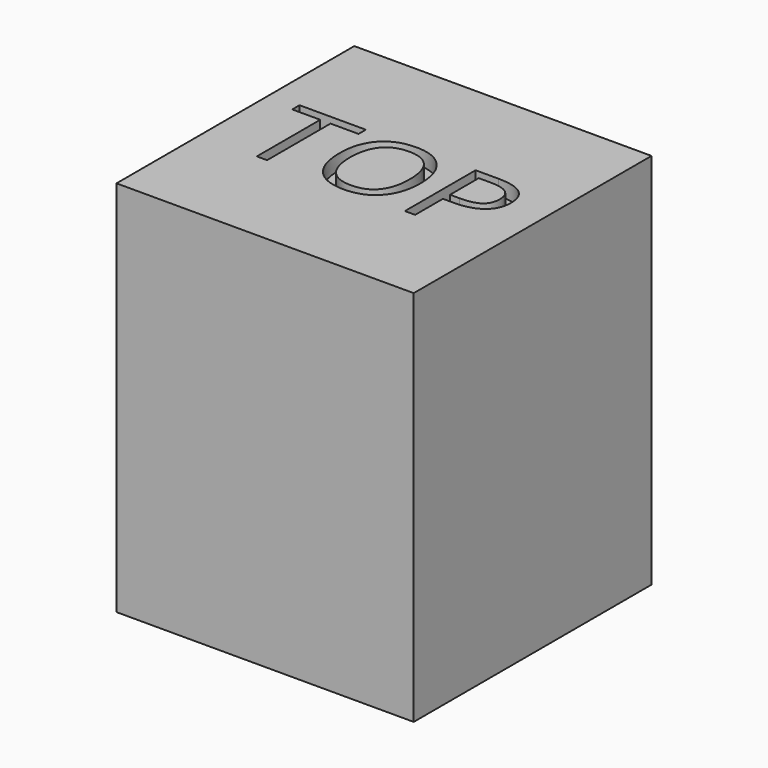
from build123d import *

# Parameters (mm, degrees)
F0_W         = 20
F0_H         = 20
F1_DEPTH     = 25.4
F2_TEXT_SIZE = 8.3333333333
F3_DEPTH     = 1


# Not quite as in the source:
# - Text() gives the source's letters only with a copy of the font that has no kerning and outlines rounded to 1/6400 em; it was checked with that copy


with BuildPart() as f1:
    # F0 (on Top) → F1 (new body)
    with BuildSketch(Plane.XY):
        Rectangle(F0_W, F0_H)
    extrude(amount=F1_DEPTH)

    # F2 (on face) → F3 (cut)
    with BuildSketch(Plane.XY.offset(25.4)):
        with Locations((-8.115234375, -3)):
            Text('TOP', F2_TEXT_SIZE, font='Open Sans', text_align=(TextAlign.LEFT, TextAlign.BOTTOM))
    extrude(amount=-F3_DEPTH, mode=Mode.SUBTRACT)


solid = f1.part
